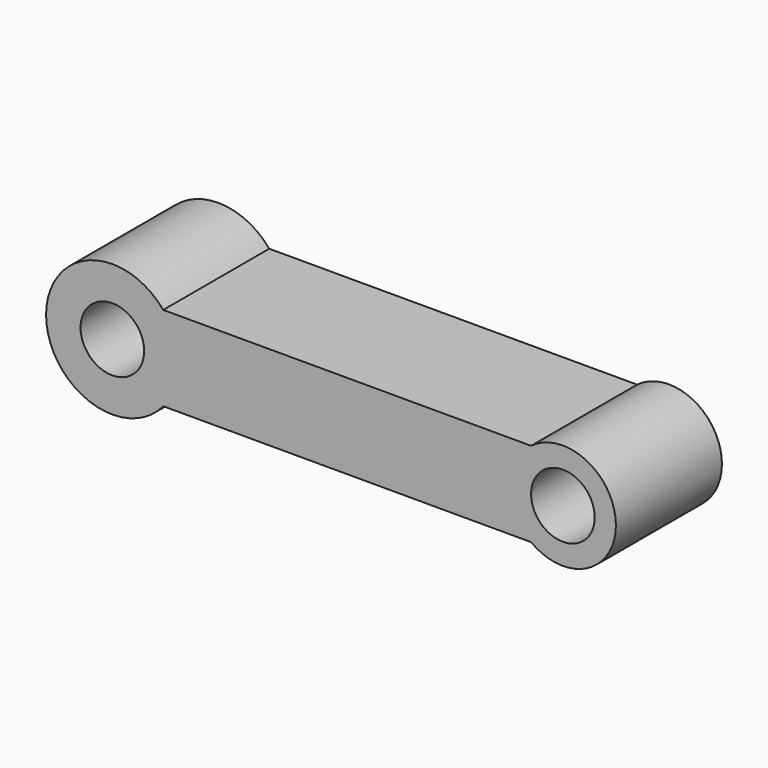
from build123d import *

# Parameters (mm, degrees)
F0_R     = 6
F1_DEPTH = 25


# Not quite as in the source:
# - a feature of the source that left no trace in its solid (it failed there, or was rolled back) is left out


with BuildPart() as f1:
    # F0 (on Front) → F1 (new body)
    with BuildSketch(Plane.XZ):
        with BuildLine():
            ThreePointArc((-30.7096580903, -8), (-28.5604391496, -4.2539052968), (-27.8143444464, 0))
            ThreePointArc((-27.8143444464, 0), (-28.5604391496, 4.2539052968), (-30.7096580903, 8))
            ThreePointArc((-30.7096580903, 8), (-52.8143444464, 0), (-30.7096580903, -8))
        make_face()
        with Locations((-40.3143444464, 0)):
            Circle(F0_R, mode=Mode.SUBTRACT)
        with BuildLine():
            ThreePointArc((-30.7096580903, 8), (-28.5604391496, 4.2539052968), (-27.8143444464, 0))
            ThreePointArc((-27.8143444464, 0), (-28.5604391496, -4.2539052968), (-30.7096580903, -8))
            Line((-30.7096580903, -8), (38.6856555536, -8))
            ThreePointArc((38.6856555536, -8), (34.6856555536, 0), (38.6856555536, 8))
            Line((38.6856555536, 8), (-30.7096580903, 8))
        make_face()
        with BuildLine():
            ThreePointArc((54.6856555536, 0), (49.1577915086, 8.94427191), (38.6856555536, 8))
            ThreePointArc((38.6856555536, 8), (34.6856555536, 0), (38.6856555536, -8))
            ThreePointArc((38.6856555536, -8), (49.1577915086, -8.94427191), (54.6856555536, 0))
        make_face()
        with Locations((44.6856555536, 0)):
            Circle(F0_R, mode=Mode.SUBTRACT)
    extrude(amount=F1_DEPTH)


solid = f1.part
